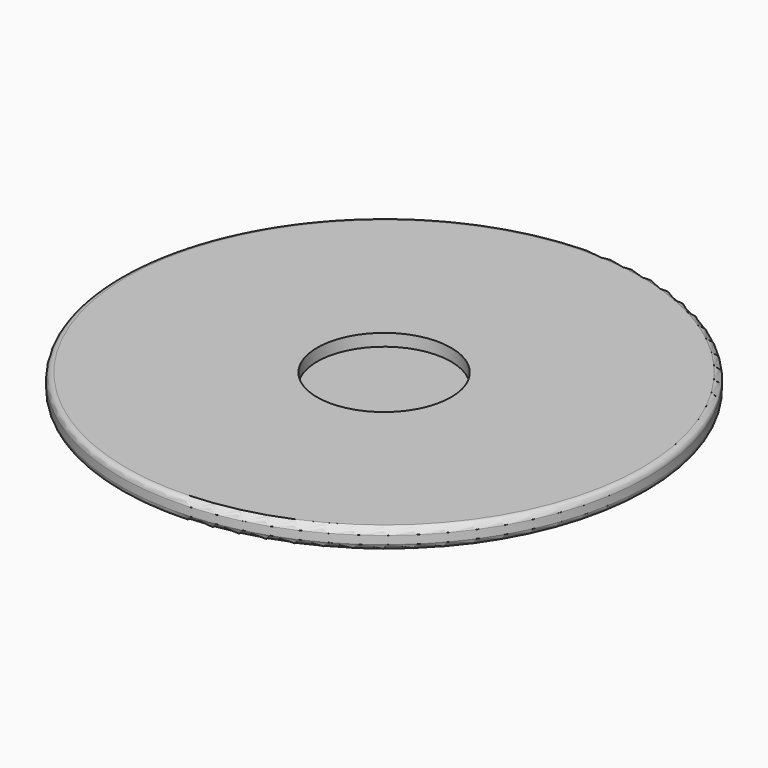
from build123d import *

# Parameters (mm, degrees)
F0_R     = 6.5
F1_DEPTH = 0.5
F2_R     = 0.15
F3_R     = 1.65
F4_DEPTH = 0.3


# Not quite as in the source:
# - a feature names something its author has since deleted; it is built from what else it names


with BuildPart() as f1:
    # F0 (on Top) → F1 (new body)
    with BuildSketch(Plane.XY):
        Circle(F0_R)
    extrude(amount=F1_DEPTH)

    # F2
    f2_edges = [f1.edges().sort_by_distance(p)[0] for p in [
        (-6.5, 0, 0.5),
        (-6.5, 0, 0),
    ]]
    fillet(f2_edges, radius=F2_R)

    # F3 (on face) → F4 (cut)
    with BuildSketch(Plane.XY.offset(0.5)):
        Circle(F3_R)
    extrude(amount=-F4_DEPTH, mode=Mode.SUBTRACT)


solid = f1.part
